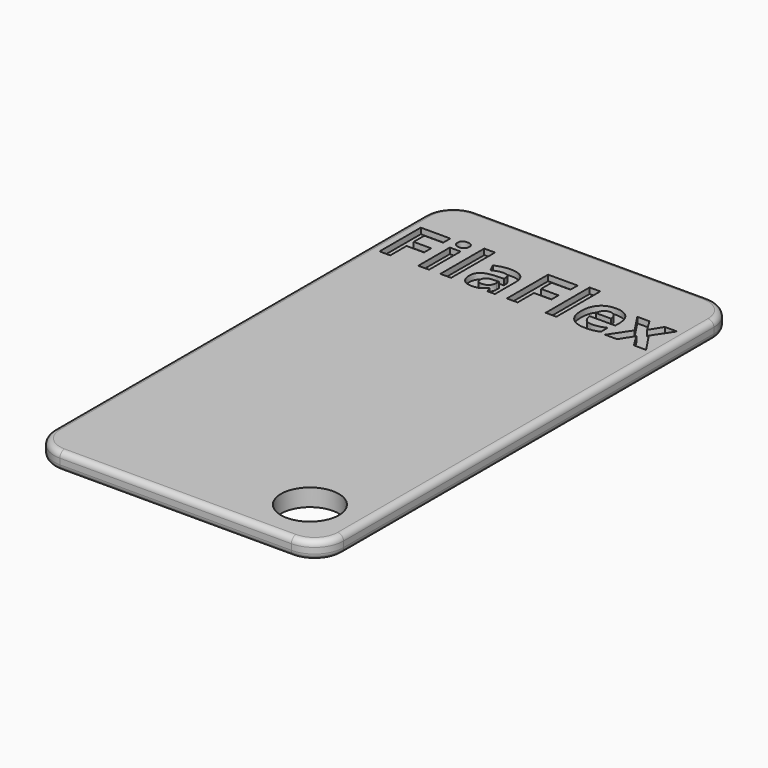
from build123d import *

# Parameters (mm, degrees)
F0_W         = 90
F0_H         = 50
F1_DEPTH     = 3
F2_R         = 1
F3_T1_DEPTH  = 3
F3_T4_ANGLE  = 90
F3_T6_ANGLE  = 90
F3_T8_ANGLE  = 90
F3_T10_ANGLE = 90
F3_T12_ANGLE = 90
F3_T14_ANGLE = 90
F3_T16_ANGLE = 90
F3_T18_ANGLE = 90
F5_ANGLE     = 90
F6_TEXT_SIZE = 12.4796880078
F7_DEPTH     = 1
F8_R         = 5
F9_DEPTH     = 3


# Not quite as in the source:
# - a fillet or chamfer that OpenCascade refuses, or shapes differently, is made with other operations: its cross-section is extruded or revolved along the edge and cut away or added
# - Text() gives the source's letters only with a copy of the font that has no kerning and outlines rounded to 1/6400 em; it was checked with that copy


with BuildPart() as f1:
    # F0 (on Top) → F1 (new body)
    with BuildSketch(Plane.XY):
        Rectangle(F0_W, F0_H)
    extrude(amount=F1_DEPTH)

    # F2
    f2_edges = [f1.edges().sort_by_distance(p)[0] for p in [
        (0, 25, 3),
        (-45, 0, 3),
        (0, -25, 3),
        (45, 0, 3),
        (0, 25, 0),
        (-45, 0, 0),
        (0, -25, 0),
        (45, 0, 0),
    ]]
    fillet(f2_edges, radius=F2_R)

    # F3: fillet of radius 5 on 4 edges, made by hand

    # F3_s2 → F3_t1 (cut)
    with BuildSketch(Plane.XY):
        with BuildLine():
            ThreePointArc((45, -20), (43.5355339059, -23.5355339059), (40, -25))
            Line((40, -25), (45, -25))
            Line((45, -25), (45, -20))
        make_face()
        with BuildLine():
            ThreePointArc((40, 25), (43.5355339059, 23.5355339059), (45, 20))
            Line((45, 20), (45, 25))
            Line((45, 25), (40, 25))
        make_face()
        with BuildLine():
            ThreePointArc((-40, 25), (-43.5355339059, 23.5355339059), (-45, 20))
            Line((-45, 20), (-45, 25))
            Line((-45, 25), (-40, 25))
        make_face()
        with BuildLine():
            ThreePointArc((-45, -20), (-43.5355339059, -23.5355339059), (-40, -25))
            Line((-40, -25), (-45, -25))
            Line((-45, -25), (-45, -20))
        make_face()
    extrude(amount=F3_T1_DEPTH, mode=Mode.SUBTRACT)

    # F3_s3 → F3_t4 (revolve, cut)
    with BuildSketch(Plane.YZ.offset(-40)):
        with BuildLine():
            ThreePointArc((-24, 0), (-24.7071067812, 0.2928932188), (-25, 1))
            Line((-25, 1), (-25, 0))
            Line((-25, 0), (-24, 0))
        make_face()
    revolve(axis=Axis((-40, -20, 0), (0, 0, -1)), revolution_arc=F3_T4_ANGLE, mode=Mode.SUBTRACT)

    # F3_s5 → F3_t6 (revolve, cut)
    with BuildSketch(Plane.XZ.offset(20)):
        with BuildLine():
            ThreePointArc((-44, 3), (-44.7071067812, 2.7071067812), (-45, 2))
            Line((-45, 2), (-45, 3))
            Line((-45, 3), (-44, 3))
        make_face()
    revolve(axis=Axis((-40, -20, 3), (0, 0, 1)), revolution_arc=F3_T6_ANGLE, mode=Mode.SUBTRACT)

    # F3_s7 → F3_t8 (revolve, cut)
    with BuildSketch(Plane.XZ.offset(-20)):
        with BuildLine():
            ThreePointArc((-44, 0), (-44.7071067812, 0.2928932188), (-45, 1))
            Line((-45, 1), (-45, 0))
            Line((-45, 0), (-44, 0))
        make_face()
    revolve(axis=Axis((-40, 20, 0), (0, 0, -1)), revolution_arc=F3_T8_ANGLE, mode=Mode.SUBTRACT)

    # F3_s9 → F3_t10 (revolve, cut)
    with BuildSketch(Plane.YZ.offset(-40)):
        with BuildLine():
            ThreePointArc((24, 3), (24.7071067812, 2.7071067812), (25, 2))
            Line((25, 2), (25, 3))
            Line((25, 3), (24, 3))
        make_face()
    revolve(axis=Axis((-40, 20, 3), (0, 0, 1)), revolution_arc=F3_T10_ANGLE, mode=Mode.SUBTRACT)

    # F3_s11 → F3_t12 (revolve, cut)
    with BuildSketch(Plane.YZ.offset(40)):
        with BuildLine():
            ThreePointArc((24, 0), (24.7071067812, 0.2928932188), (25, 1))
            Line((25, 1), (25, 0))
            Line((25, 0), (24, 0))
        make_face()
    revolve(axis=Axis((40, 20, 0), (0, 0, -1)), revolution_arc=F3_T12_ANGLE, mode=Mode.SUBTRACT)

    # F3_s13 → F3_t14 (revolve, cut)
    with BuildSketch(Plane.XZ.offset(-20)):
        with BuildLine():
            ThreePointArc((44, 3), (44.7071067812, 2.7071067812), (45, 2))
            Line((45, 2), (45, 3))
            Line((45, 3), (44, 3))
        make_face()
    revolve(axis=Axis((40, 20, 3), (0, 0, 1)), revolution_arc=F3_T14_ANGLE, mode=Mode.SUBTRACT)

    # F3_s15 → F3_t16 (revolve, cut)
    with BuildSketch(Plane.XZ.offset(20)):
        with BuildLine():
            ThreePointArc((44, 0), (44.7071067812, 0.2928932188), (45, 1))
            Line((45, 1), (45, 0))
            Line((45, 0), (44, 0))
        make_face()
    revolve(axis=Axis((40, -20, 0), (0, 0, -1)), revolution_arc=F3_T16_ANGLE, mode=Mode.SUBTRACT)

    # F3_s17 → F3_t18 (revolve, cut)
    with BuildSketch(Plane.YZ.offset(40)):
        with BuildLine():
            ThreePointArc((-24, 3), (-24.7071067812, 2.7071067812), (-25, 2))
            Line((-25, 2), (-25, 3))
            Line((-25, 3), (-24, 3))
        make_face()
    revolve(axis=Axis((40, -20, 3), (0, 0, 1)), revolution_arc=F3_T18_ANGLE, mode=Mode.SUBTRACT)


with BuildPart() as f1_1:
    # F5: moved
    add(f1.part.rotate(Axis((0, 0, 16.4477843791), (0, 0, 1)), F5_ANGLE))

    # F6 (on face) → F7 (cut)
    with BuildSketch(Plane.XY.offset(3)):
        with Locations((-24, 27.6281953682)):
            Text('FilaFlex', F6_TEXT_SIZE, font='Open Sans', font_style=FontStyle.BOLD, text_align=(TextAlign.LEFT, TextAlign.BOTTOM))
    extrude(amount=-F7_DEPTH, mode=Mode.SUBTRACT)

    # F8 (on face) → F9 (cut)
    with BuildSketch(Plane.XY.offset(3)):
        with Locations((16, -36)):
            Circle(F8_R)
    extrude(amount=-F9_DEPTH, mode=Mode.SUBTRACT)


solid = f1_1.part
